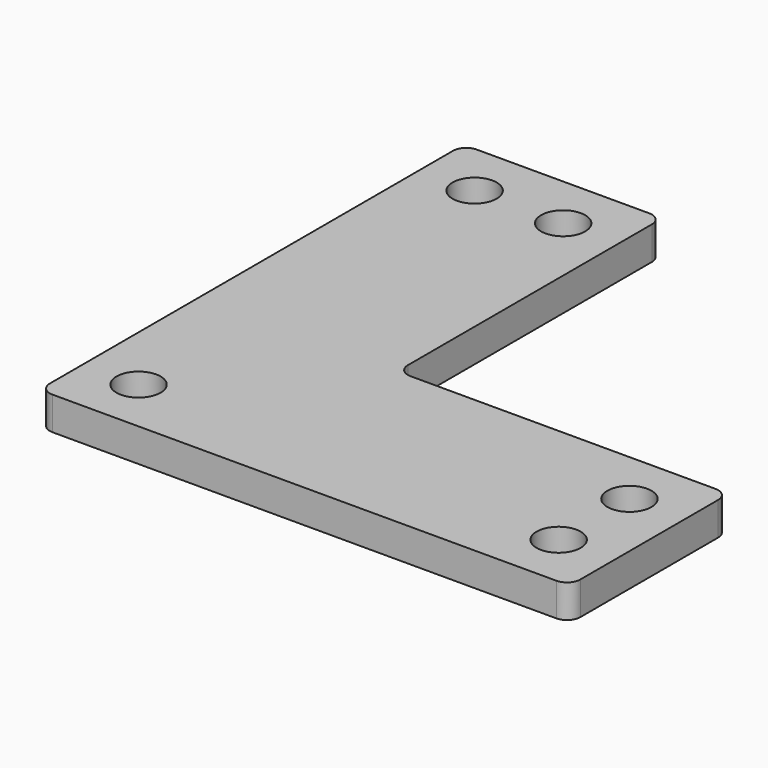
from build123d import *

# Parameters (mm, degrees)
F1_DEPTH = 6.35
F2_R     = 4.22275
F3_DEPTH = 6.351
F4_R     = 2.54


# Not quite as in the source:
# - a length typed as a fraction of an inch, garbled in the dataset ("3 / 203.2 mm" for 3/8 in), is restored


with BuildPart() as f1:
    # F0 (on Top) → F1 (new body)
    with BuildSketch(Plane.XY):
        Polygon((0, 78.937935479), (-38.1, 78.937935479), (-38.1, -22.662064521), (63.5, -22.662064521), (63.5, 15.437935479), (0, 15.437935479), align=None)
    extrude(amount=F1_DEPTH)

    # F2 (on face) → F3 (cut, through all)
    with BuildSketch(Plane.XY.offset(6.35)):
        with Locations((-27.52725, 68.365185479)):
            Circle(F2_R)
        with Locations((-10.57275, 68.365185479)):
            Circle(F2_R)
        with Locations((52.92725, 4.865185479)):
            Circle(F2_R)
        with Locations((52.92725, -12.089314521)):
            Circle(F2_R)
        with Locations((-27.52725, -12.089314521)):
            Circle(F2_R)
    extrude(amount=-F3_DEPTH, mode=Mode.SUBTRACT)

    # F4
    f4_edges = [f1.edges().sort_by_distance(p)[0] for p in [
        (-38.1, -22.662065, 3.175),
        (63.5, -22.662065, 3.175),
        (63.5, 15.437935, 3.175),
        (0, 15.437935, 3.175),
        (0, 78.937935, 3.175),
        (-38.1, 78.937935, 3.175),
    ]]
    fillet(f4_edges, radius=F4_R)


solid = f1.part
